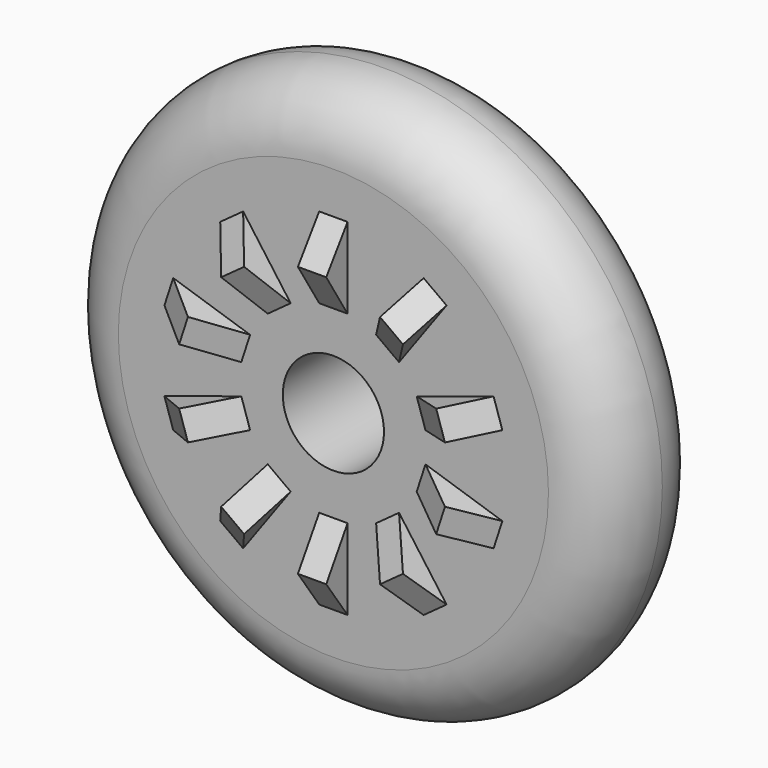
from build123d import *

# Parameters (mm, degrees)
F0_R     = 6.985
F0_R_2   = 1.27
F1_DEPTH = 1.5875
F2_R     = 1.58749
F4_DEPTH = 0.3556
F5_COUNT = 10


# Not quite as in the source:
# - a fillet or chamfer is up to 0.001 mm smaller than in the source, because OpenCascade refuses the exact size


with BuildPart() as f1:
    # F0 (on Front) → F1 (new body, symmetric)
    with BuildSketch(Plane.XZ):
        Circle(F0_R)
        Circle(F0_R_2, mode=Mode.SUBTRACT)
    extrude(amount=F1_DEPTH, both=True)

    # F2 (radius 1.5875 in the source; OpenCascade refuses exactly that, so slightly less here)
    f2_edges = [f1.edges().sort_by_distance(p)[0] for p in [
        (-6.985, 1.5875, 0),
        (-6.985, -1.5875, 0),
    ]]
    fillet(f2_edges, radius=F2_R)

    # F3 (on Right) → F4 (join, symmetric)
    with BuildSketch(Plane.YZ):
        Polygon((-1.5832948266, 2.3071307223), (-1.4941976026, 4.4750159141), (-2.2568043449, 3.3910733182), align=None)
    f4 = extrude(amount=F4_DEPTH, both=True)

    # F5: F4 ×10 about axis
    f5_axis = Axis((0, -1.5875, 0), (0, -1, 0))
    for i in range(1, F5_COUNT):
        add(f4.rotate(f5_axis, i * 360 / F5_COUNT))


solid = f1.part
